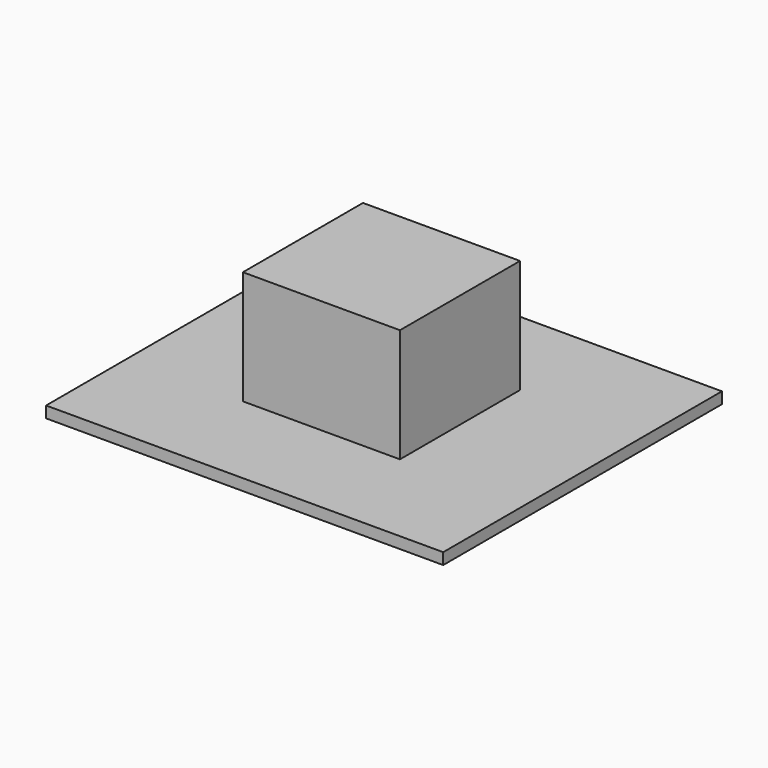
from build123d import *

# Parameters (mm, degrees)
F0_W        = 104.8084236681
F0_H        = 91.941319406
F1_DEPTH    = 3
F2_W        = 41.4473675191
F2_H        = 39.6052636206
F3_DEPTH    = 30
F4_T        = 3
F4_T3_DEPTH = 47.4473675191
F4_T5_DEPTH = 45.6052636206


# Not quite as in the source:
# - a shell that OpenCascade refuses in one call is made with other operations: the cavity is built on its own and cut out


with BuildPart() as f1:
    # F0 (on Top) → F1 (new body)
    with BuildSketch(Plane.XY):
        with Locations((0.5848687142, -2.3394748569)):
            Rectangle(F0_W, F0_H)
    extrude(amount=F1_DEPTH)

    # F2 (on face) → F3 (join)
    with BuildSketch(Plane.XY.offset(3)):
        with Locations((-0.575657934, -1.7269738019)):
            Rectangle(F2_W, F2_H)
    extrude(amount=F3_DEPTH)

    # F4: shell of thickness 3, made by hand


with BuildPart() as f4_core1:
    # F4_t2: copy of F1
    add(f1.part)

    # the walls: a layer under each face that stays
    f4_faces = [f4_core1.faces().sort_by_distance(p)[0] for p in [
        (0.5848687142, 43.6311848462, 1.5),
        (52.9890805483, -2.3394748569, 1.5),
        (-51.8193431199, -2.3394748569, 1.5),
        (-34.3512725085, -32.9865813255, 3),
        (0.5848687142, -48.3101345599, 1.5),
        (-0.575657934, 18.0756580085, 18),
        (-21.2993416935, -1.7269738019, 18),
        (-0.575657934, -21.5296056122, 18),
        (20.1480258256, -1.7269738019, 18),
        (-0.575657934, -1.7269738019, 33),
    ]]
    thicken(f4_faces, amount=-F4_T, mode=Mode.SUBTRACT)

    # F4_s4 → F4_t3 (cut)
    with BuildSketch(Plane.YZ.offset(-24.2993416935)):
        Polygon((18.1056580085, 3.03), (18.0756580085, 0), (15.0756580085, 0), (15.0756580085, 3), align=None)
        Polygon((-21.5596056122, 3.03), (-21.5296056122, 0), (-18.5296056122, 0), (-18.5296056122, 3), align=None)
    extrude(amount=F4_T3_DEPTH, mode=Mode.SUBTRACT)

    # F4_s6 → F4_t5 (cut)
    with BuildSketch(Plane.XZ.offset(-21.0756580085)):
        Polygon((-21.3293416935, 3.03), (-21.2993416935, 0), (-18.2993416935, 0), (-18.2993416935, 3), align=None)
        Polygon((20.1780258256, 3.03), (20.1480258256, 0), (17.1480258256, 0), (17.1480258256, 3), align=None)
    extrude(amount=F4_T5_DEPTH, mode=Mode.SUBTRACT)


with BuildPart() as f1_1:
    add(f1.part)

    # what is left inside the walls is the cavity
    f4_cavity = [f4_core1.part.solids().sort_by_distance(p)[0] for p in [
        (-0.575658, -7.327851, 0.03),
    ]]
    add(f4_cavity, mode=Mode.SUBTRACT)


solid = f1_1.part
